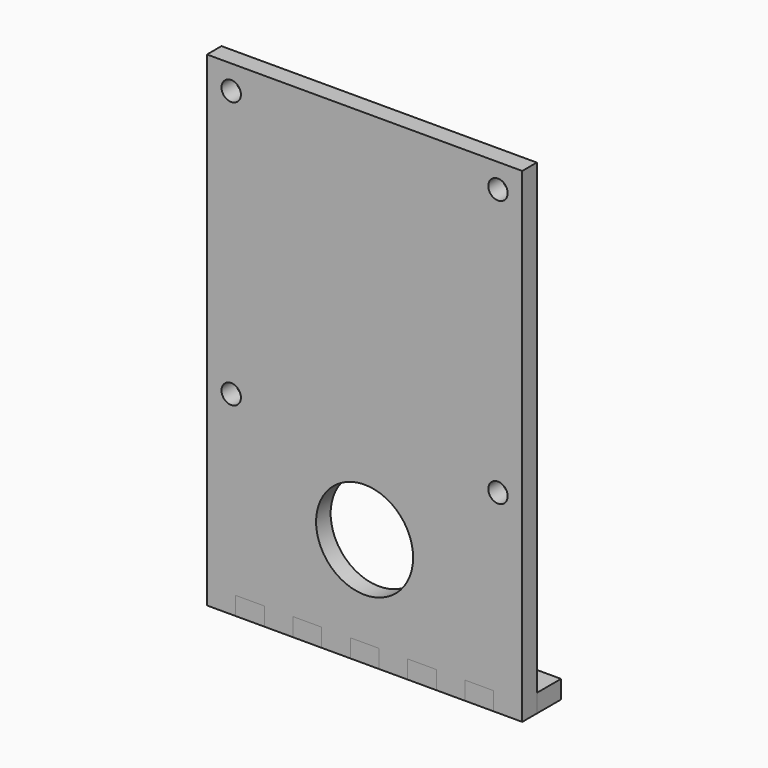
from build123d import *

# Parameters (mm, degrees)
F0_R     = 1.6
F0_R_2   = 8
F1_DEPTH = 3
F2_W     = 4.7272727273
F2_H     = 3
F3_DEPTH = 8


# Not quite as in the source:
# - a feature names something its author has since deleted; it is built from what else it names


with BuildPart() as f1:
    # F0 (on Front) → F1 (new body)
    with BuildSketch(Plane.XZ):
        Polygon((0, 80), (0, 0), (4.7272727273, 0), (4.7272727273, 3), (9.4545454545, 3), (9.4545454545, 0), (14.1818181818, 0), (14.1818181818, 3), (18.9090909091, 3), (18.9090909091, 0), (23.6363636364, 0), (23.6363636364, 3), (28.3636363636, 3), (28.3636363636, 0), (33.0909090909, 0), (33.0909090909, 3), (37.8181818182, 3), (37.8181818182, 0), (42.5454545455, 0), (42.5454545455, 3), (47.2727272727, 3), (47.2727272727, 0), (52, 0), (52, 80), align=None)
        with Locations((4, 32)):
            Circle(F0_R, mode=Mode.SUBTRACT)
        with Locations((26, 18)):
            Circle(F0_R_2, mode=Mode.SUBTRACT)
        with Locations((48, 32)):
            Circle(F0_R, mode=Mode.SUBTRACT)
        with Locations((4, 76)):
            Circle(F0_R, mode=Mode.SUBTRACT)
        with Locations((48, 76)):
            Circle(F0_R, mode=Mode.SUBTRACT)
    extrude(amount=F1_DEPTH)


with BuildPart() as f3:
    # F2 (on face) → F3 (new body)
    with BuildSketch(Plane.XZ.offset(3)):
        with Locations((2.3636363636, 1.5)):
            Rectangle(F2_W, F2_H)
        with Locations((7.0909090909, 1.5)):
            Rectangle(F2_W, F2_H)
        with Locations((11.8181818182, 1.5)):
            Rectangle(F2_W, F2_H)
        with Locations((16.5454545455, 1.5)):
            Rectangle(F2_W, F2_H)
        with Locations((21.2727272727, 1.5)):
            Rectangle(F2_W, F2_H)
        with Locations((26, 1.5)):
            Rectangle(F2_W, F2_H)
        with Locations((30.7272727273, 1.5)):
            Rectangle(F2_W, F2_H)
        with Locations((35.4545454545, 1.5)):
            Rectangle(F2_W, F2_H)
        with Locations((40.1818181818, 1.5)):
            Rectangle(F2_W, F2_H)
        with Locations((44.9090909091, 1.5)):
            Rectangle(F2_W, F2_H)
        with Locations((49.6363636364, 1.5)):
            Rectangle(F2_W, F2_H)
    extrude(amount=-F3_DEPTH)

    # F4: cut F1
    add(f1.part, mode=Mode.SUBTRACT)


solid = Compound([f1.part, f3.part])
